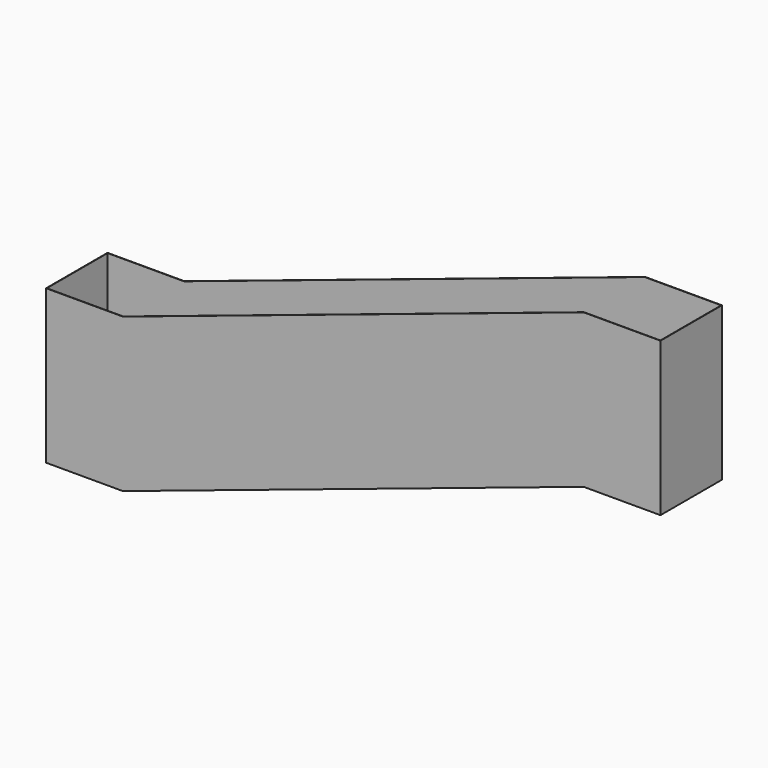
from build123d import *

# Parameters (mm, degrees)
F1_DEPTH = 200
F2_T     = -1
F6_D     = 20
F7_D     = 20


# Not quite as in the source:
# - the program builds the solid bodies; features that only make, move or delete a surface that nothing else refers to are left out


with BuildPart() as f1:
    # F0 (on Front) → F1 (new body)
    with BuildSketch(Plane.XZ):
        Polygon((0, 400), (0, 0), (200, 0), (1400, 400), (1600, 400), (1600, 800), (1400, 800), (200, 400), align=None)
    extrude(amount=F1_DEPTH)

    # F2
    f2_openings = [f1.faces().sort_by_distance(p)[0] for p in [
        (100, -100, 400),
        (1500, -100, 800),
        (800, -100, 600),
    ]]
    offset(amount=F2_T, openings=f2_openings, kind=Kind.INTERSECTION)

    # F6 (through all)
    with Locations(Plane.XY.offset(401)):
        with Locations((13, -187), (13, -13)):
            Hole(F6_D / 2)

    # F7 (through all)
    with Locations(Plane.XY.offset(401)):
        with Locations((1587, -13), (1587, -187)):
            Hole(F7_D / 2)


solid = f1.part
